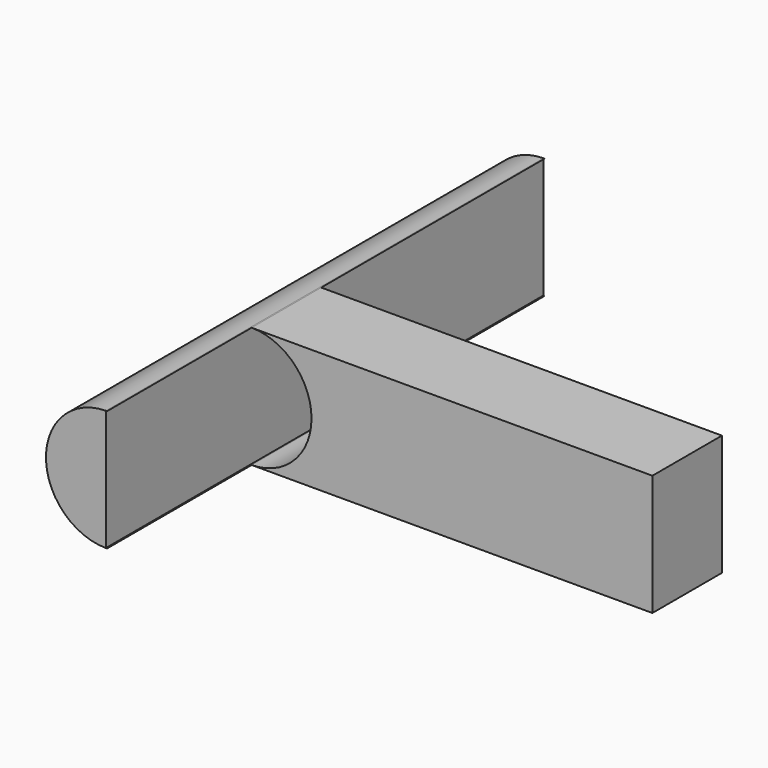
from build123d import *

# Parameters (mm, degrees)
F1_DEPTH      = 77
F1_DEPTH_BACK = 80.3
F2_DEPTH      = 25


with BuildPart() as f1:
    # F0 (on Front) → F1 (new body, two sides)
    with BuildSketch(Plane.XZ) as f1_sk:
        with BuildLine():
            Line((-3.9150179645, -8.5844577717), (-3.9150179645, 26.1770182716))
            ThreePointArc((-3.9150179645, 26.1770182716), (-21.1170714481, 8.79628025), (-3.9150179645, -8.5844577717))
        make_face()
    extrude(amount=F1_DEPTH)
    extrude(f1_sk.sketch, amount=-F1_DEPTH_BACK)


with BuildPart() as f1b:
    # F0 (on Front) → F1, piece 2 (new body, two sides)
    with BuildSketch(Plane.XZ) as f1_2_sk:
        with BuildLine():
            ThreePointArc((-3.5557928214, 26.1770182716), (-3.7354053929, 26.1779463051), (-3.9150179645, 26.1770182716))
            Line((-3.9150179645, 26.1770182716), (-3.5557928214, 26.1770182716))
        make_face()
    extrude(amount=F1_DEPTH)
    extrude(f1_2_sk.sketch, amount=-F1_DEPTH_BACK)


with BuildPart() as f1c:
    # F0 (on Front) → F1, piece 3 (new body, two sides)
    with BuildSketch(Plane.XZ) as f1_3_sk:
        with BuildLine():
            Line((-3.5557928214, -8.5844577717), (-3.9150179645, -8.5844577717))
            ThreePointArc((-3.9150179645, -8.5844577717), (-3.7354053929, -8.5853858052), (-3.5557928214, -8.5844577717))
        make_face()
    extrude(amount=F1_DEPTH)
    extrude(f1_3_sk.sketch, amount=-F1_DEPTH_BACK)


with BuildPart() as f2:
    # F0 (on Front) → F2 (new body)
    with BuildSketch(Plane.XZ):
        with BuildLine():
            Line((111.6774268448, 26.1770182716), (-3.5557928214, 26.1770182716))
            ThreePointArc((-3.5557928214, 26.1770182716), (8.6186279685, 21.0233066488), (13.6462606622, 8.79628025))
            ThreePointArc((13.6462606622, 8.79628025), (8.6186279685, -3.4307461489), (-3.5557928214, -8.5844577717))
            Line((-3.5557928214, -8.5844577717), (111.6774268448, -8.5844577717))
            Line((111.6774268448, -8.5844577717), (111.6774268448, 26.1770182716))
        make_face()
    extrude(amount=F2_DEPTH)


solid = Compound([f1.part, f1b.part, f1c.part, f2.part])
